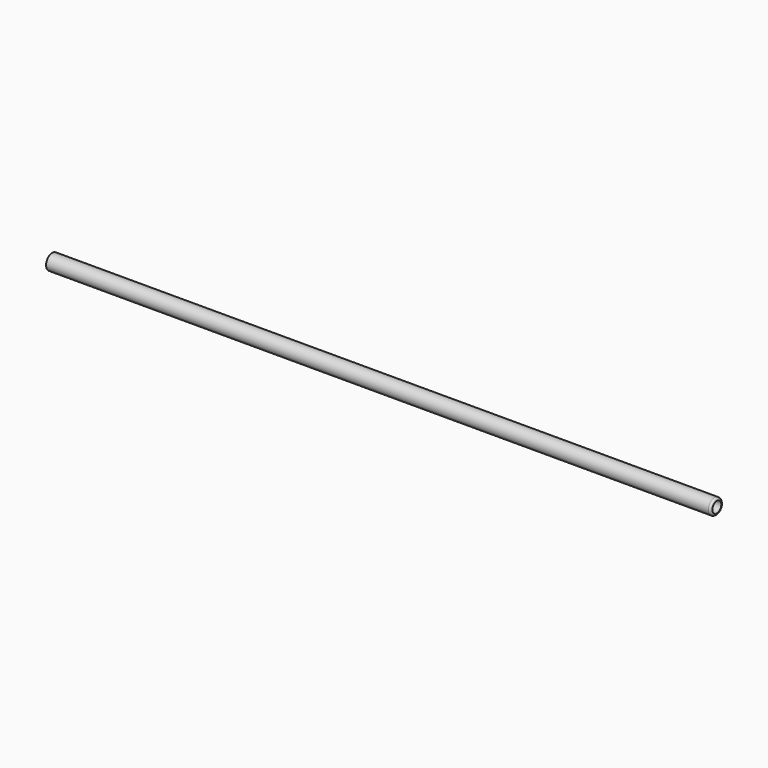
from build123d import *

# Parameters (mm, degrees)
F0_R     = 3.5
F0_R_2   = 2.5
F1_DEPTH = 300
F2_R     = 0.99999


# Not quite as in the source:
# - a fillet or chamfer is up to 0.001 mm smaller than in the source, because OpenCascade refuses the exact size


with BuildPart() as f1:
    # F0 (on Right) → F1 (new body)
    with BuildSketch(Plane.YZ):
        Circle(F0_R)
        Circle(F0_R_2, mode=Mode.SUBTRACT)
    extrude(amount=F1_DEPTH)

    # F2 (radius 1 in the source; OpenCascade refuses exactly that, so slightly less here)
    f2_edges = [f1.edges().sort_by_distance(p)[0] for p in [
        (300, -3.5, 0),
    ]]
    fillet(f2_edges, radius=F2_R)


solid = f1.part
